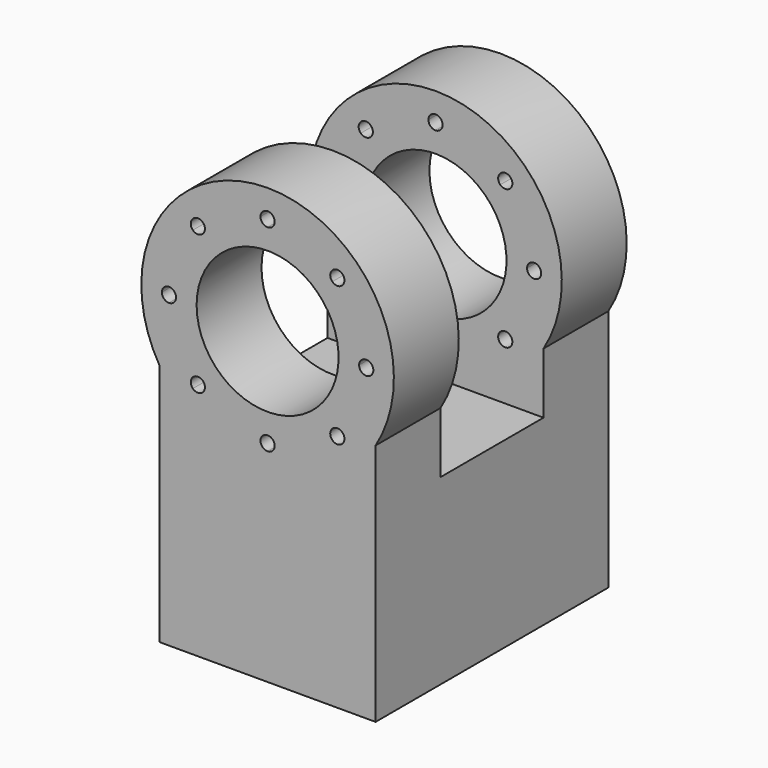
from build123d import *

# Parameters (mm, degrees)
F0_W             = 53.254
F0_H             = 20
F0_H_2           = 31.75
F1_DEPTH         = 45
F2_W             = 53.254
F2_H             = 20
F3_DEPTH         = 15
F4_R             = 31.1332376333
F5_DEPTH         = 20
F6_R             = 31.1332376333
F7_DEPTH         = 20
F8_R             = 17.5
F9_DEPTH         = 100
F11_DEPTH        = 100
F11_COPIES_COUNT = 8


# Not quite as in the source:
# - a pattern or mirror of a feature is missing from the dataset's text; its kind, count and spacing are read off the source's solid


with BuildPart() as f1:
    # F0 (on Top) → F1 (new body)
    with BuildSketch(Plane.XY):
        with Locations((0, 25.875)):
            Rectangle(F0_W, F0_H)
        Rectangle(F0_W, F0_H_2)
        with Locations((0, -25.875)):
            Rectangle(F0_W, F0_H)
    extrude(amount=F1_DEPTH)

    # F2 (on face) → F3 (join)
    with BuildSketch(Plane.XY.offset(45)):
        with Locations((0, 25.875)):
            Rectangle(F2_W, F2_H)
        with Locations((0, -25.875)):
            Rectangle(F2_W, F2_H)
    extrude(amount=F3_DEPTH)

    # F4 (on face) → F5 (join)
    with BuildSketch(Plane.XZ.offset(-15.875)):
        with Locations((0, 76.1332376333)):
            Circle(F4_R)
    extrude(amount=-F5_DEPTH)

    # F6 (on face) → F7 (join)
    with BuildSketch(Plane(origin=(0, -15.875, 0), x_dir=(-1, 0, 0), z_dir=(0, 1, 0))):
        with Locations((0, 76.1332376333)):
            Circle(F6_R)
    extrude(amount=-F7_DEPTH)

    # F8 (on face) → F9 (cut)
    with BuildSketch(Plane(origin=(0, 35.875, 0), x_dir=(-1, 0, 0), z_dir=(0, 1, 0))):
        with Locations((0, 76.1332376333)):
            Circle(F8_R)
    extrude(amount=-F9_DEPTH, mode=Mode.SUBTRACT)

    # F10 (on face) → F11 (cut)
    with BuildSketch(Plane(origin=(0, 35.875, 0), x_dir=(-1, 0, 0), z_dir=(0, 1, 0))):
        with BuildLine():
            ThreePointArc((0, 102.19985645), (-1.75, 100.44985645), (0, 98.69985645))
            Line((0, 98.69985645), (0, 102.19985645))
        make_face()
        with BuildLine():
            Line((0, 102.19985645), (0, 98.69985645))
            ThreePointArc((0, 98.69985645), (1.2374368671, 99.2124195829), (1.75, 100.44985645))
            ThreePointArc((1.75, 100.44985645), (1.2374368671, 101.6872933171), (0, 102.19985645))
        make_face()
    f11 = extrude(amount=-F11_DEPTH, mode=Mode.SUBTRACT)

    # F11_copies: F11 ×8 about axis
    f11_copies_axis = Axis((0, 0, 76.133238), (0, 1, 0))
    for i in range(1, F11_COPIES_COUNT):
        add(f11.rotate(f11_copies_axis, i * 360 / F11_COPIES_COUNT), mode=Mode.SUBTRACT)


solid = f1.part
